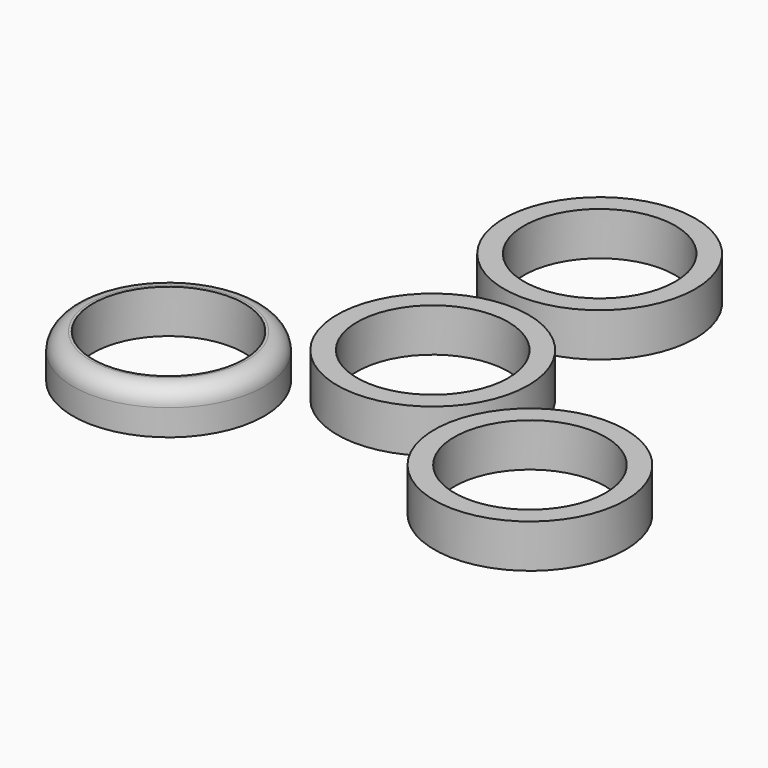
from build123d import *

# Parameters (mm, degrees)
F0_R     = 13.97
F0_R_2   = 11.049
F2_DEPTH = 6.35
F4_R     = 2.54


# Not quite as in the source:
# - a feature of the source that left no trace in its solid (it failed there, or was rolled back) is left out


with BuildPart() as f2:
    # F0 (on Top) → F2 (new body)
    with BuildSketch(Plane.XY):
        with Locations((0, 30.48)):
            Circle(F0_R)
        with Locations((0, 30.48)):
            Circle(F0_R_2, mode=Mode.SUBTRACT)
    extrude(amount=F2_DEPTH)


with BuildPart() as f2b:
    # F0 (on Top) → F2, piece 2 (new body)
    with BuildSketch(Plane.XY):
        Circle(F0_R)
        Circle(F0_R_2, mode=Mode.SUBTRACT)
    extrude(amount=F2_DEPTH)


with BuildPart() as f2c:
    # F0 (on Top) → F2, piece 3 (new body)
    with BuildSketch(Plane.XY):
        with Locations((26.3964543073, -15.24)):
            Circle(F0_R)
        with Locations((26.3964543073, -15.24)):
            Circle(F0_R_2, mode=Mode.SUBTRACT)
    extrude(amount=F2_DEPTH)


with BuildPart() as f2d:
    # F0 (on Top) → F2, piece 4 (new body)
    with BuildSketch(Plane.XY):
        with Locations((-26.3964543073, -15.24)):
            Circle(F0_R)
        with Locations((-26.3964543073, -15.24)):
            Circle(F0_R_2, mode=Mode.SUBTRACT)
    extrude(amount=F2_DEPTH)

    # F4
    f4_edges = [f2d.edges().sort_by_distance(p)[0] for p in [
        (-40.366454, -15.24, 6.35),
    ]]
    fillet(f4_edges, radius=F4_R)


solid = Compound([f2.part, f2b.part, f2c.part, f2d.part])
